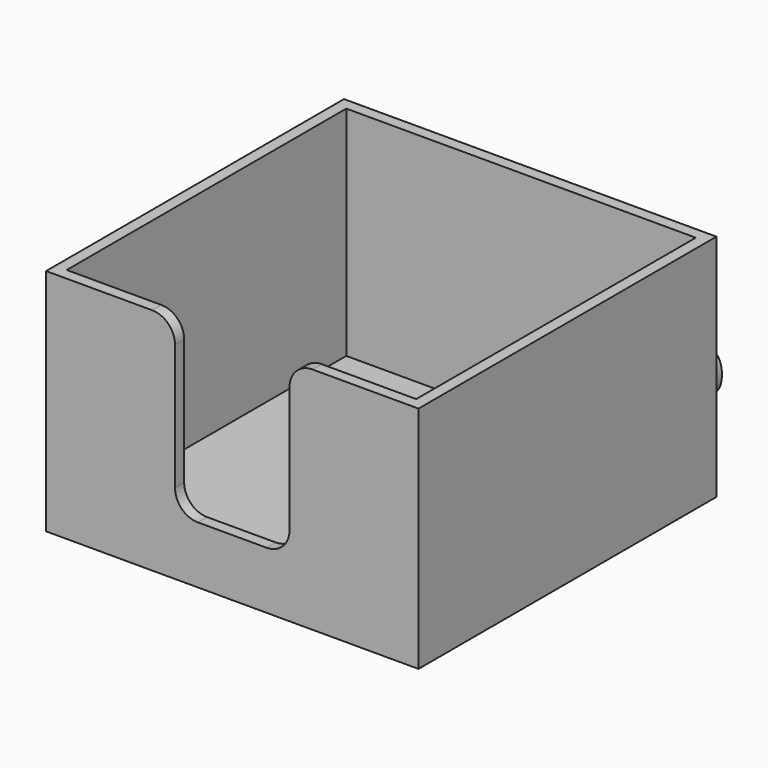
from build123d import *

# Parameters (mm, degrees)
F0_W         = 82.55
F0_H         = 82.55
F1_DEPTH     = 50.8
F2_T         = -2.54
F3_W         = 12.7
F3_H         = 38.1
F4_DEPTH     = 25.4
F5_R         = 5.08
F6_TEXT_SIZE = 13.2301605189
F7_DEPTH     = 2.54


# Not quite as in the source:
# - Text() gives the source's letters only with a copy of the font that has no kerning and outlines rounded to 1/6400 em; it was checked with that copy


with BuildPart() as f1:
    # F0 (on Top) → F1 (new body)
    with BuildSketch(Plane.XY):
        Rectangle(F0_W, F0_H)
    extrude(amount=F1_DEPTH)

    # F2
    f2_openings = [f1.faces().sort_by_distance(p)[0] for p in [
        (0, 0, 50.8),
    ]]
    offset(amount=F2_T, openings=f2_openings)

    # F3 (on face) → F4 (cut)
    with BuildSketch(Plane.XZ.offset(41.275)):
        with Locations((-6.35, 31.75)):
            Rectangle(F3_W, F3_H)
        with Locations((6.35, 31.75)):
            Rectangle(F3_W, F3_H)
    extrude(amount=-F4_DEPTH, mode=Mode.SUBTRACT)

    # F5
    f5_edges = [f1.edges().sort_by_distance(p)[0] for p in [
        (-12.7, -40.005, 50.8),
        (12.7, -40.005, 50.8),
        (12.7, -40.005, 12.7),
        (-12.7, -40.005, 12.7),
    ]]
    fillet(f5_edges, radius=F5_R)

    # F6 (on face) → F7 (join)
    with BuildSketch(Plane(origin=(0, 41.275, 0), x_dir=(-1, 0, 0), z_dir=(0, 1, 0))):
        with Locations((-41.275, 17.820584521)):
            Text('Orcas Vikings', F6_TEXT_SIZE, font='Open Sans', text_align=(TextAlign.LEFT, TextAlign.BOTTOM))
    extrude(amount=F7_DEPTH)


solid = f1.part
